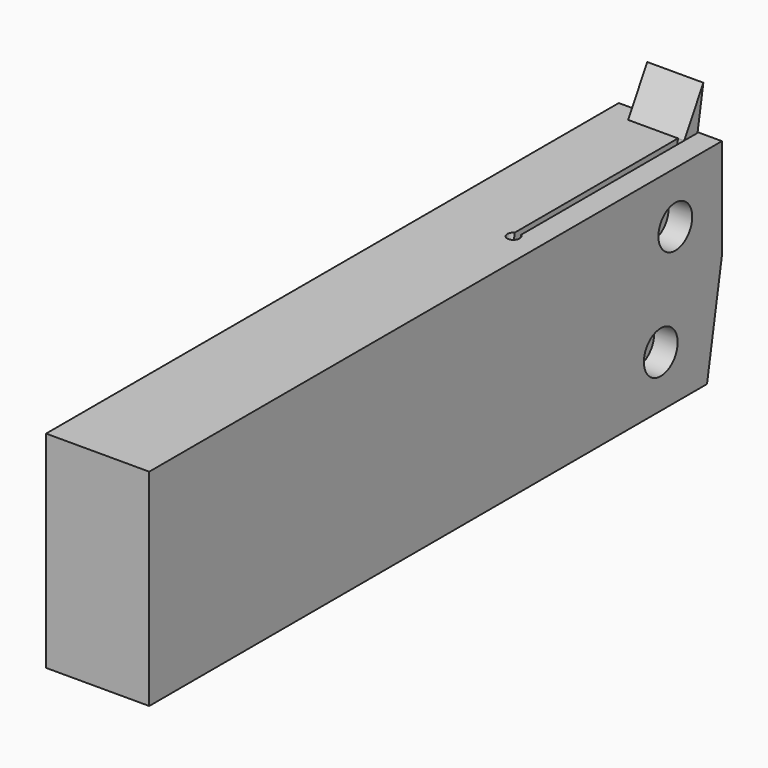
from build123d import *

# Parameters (mm, degrees)
F1_DEPTH      = 6.9088
F0_R          = 2.6
F0_R_2        = 2.1
F2_DEPTH      = 9.8044
F2_DEPTH_BACK = 2.8956
F4_DEPTH      = 31.751
F4_DEPTH_BACK = 14.4809433496
F5_R          = 2.6
F5_R_2        = 2.1
F6_DEPTH      = 3.6576


with BuildPart() as f1:
    # F0 (on Right) → F1 (new body)
    with BuildSketch(Plane.YZ):
        Polygon((7.325553628, -30.48), (11.804258938, -5.08), (9.7670606325, -5.08), (9.7479808874, -5.113047088), (5.2751026706, -30.48), align=None)
        Polygon((11.804258938, -5.08), (12.7, 0), (9.7670606325, -5.08), align=None)
        Polygon((7.1866703591, -31.2676461581), (7.325553628, -30.48), (5.2751026706, -30.48), (5.1980480634, -30.916998393), align=None)
    extrude(amount=F1_DEPTH)


with BuildPart() as f2:
    # F0 (on Right) → F2 (new body, two sides)
    with BuildSketch(Plane.YZ) as f2_sk:
        Polygon((11.938, -5.08), (11.804258938, -5.08), (7.325553628, -30.48), (9.6468188628, -30.48), (11.938, -17.486066071), align=None)
        Polygon((7.325553628, -30.48), (11.804258938, -5.08), (9.7670606325, -5.08), (9.7479808874, -5.113047088), (5.2751026706, -30.48), align=None)
        Polygon((9.7479808874, -5.113047088), (9.7670606325, -5.08), (-76.2, -5.08), (-76.2, -30.48), (5.2751026706, -30.48), align=None)
        with Locations((2.5260036068, -24.13)):
            Circle(F0_R, mode=Mode.SUBTRACT)
        with Locations((4.7653562618, -11.43)):
            Circle(F0_R, mode=Mode.SUBTRACT)
        with Locations((2.5260036068, -24.13)):
            Circle(F0_R)
        with Locations((2.5260036068, -24.13)):
            Circle(F0_R_2, mode=Mode.SUBTRACT)
        with Locations((4.7653562618, -11.43)):
            Circle(F0_R)
        with Locations((4.7653562618, -11.43)):
            Circle(F0_R_2, mode=Mode.SUBTRACT)
    extrude(amount=F2_DEPTH)
    extrude(f2_sk.sketch, amount=-F2_DEPTH_BACK)

    # F3 (on face) → F4 (cut, two sides)
    with BuildSketch(Plane(origin=(0, -5.1303777829, -29.095818248), x_dir=(1, 0, 0), z_dir=(0, -0.1736481777, -0.984807753))) as f4_sk:
        Polygon((6.1468, -10.4877584633), (0, -10.4877584633), (0, -12.4816584633), (0.2903233285, -12.5070584633), (6.6184766715, -12.5070584633), (6.9088, -12.4816584633), (6.9088, -10.4877584633), align=None)
        Polygon((6.6184766715, -12.5070584633), (0.2903233285, -12.5070584633), (2.54, -12.7038796686), (2.54, -14.7930584633), (4.3688, -14.7930584633), (4.3688, -12.7038796686), align=None)
        with BuildLine():
            Line((6.1468, 14.2523301791), (6.1468, -10.4877584633))
            Line((6.1468, -10.4877584633), (6.9088, -10.4877584633))
            Line((6.9088, -10.4877584633), (6.9088, 14.2523301791))
            ThreePointArc((6.9088, 14.2523301791), (6.5278, 15.6742415367), (6.1468, 14.2523301791))
        make_face()
    extrude(amount=-F4_DEPTH, mode=Mode.SUBTRACT)
    extrude(f4_sk.sketch, amount=F4_DEPTH_BACK, mode=Mode.SUBTRACT)

    # F5 (on face) → F6 (cut, through all)
    with BuildSketch(Plane.YZ.offset(6.1468)):
        with Locations((4.7653562618, -11.43)):
            Circle(F5_R)
        with Locations((4.7653562618, -11.43)):
            Circle(F5_R_2, mode=Mode.SUBTRACT)
        with Locations((2.5260036068, -24.13)):
            Circle(F5_R)
        with Locations((2.5260036068, -24.13)):
            Circle(F5_R_2, mode=Mode.SUBTRACT)
    extrude(amount=F6_DEPTH, mode=Mode.SUBTRACT)


solid = Compound([f1.part, f2.part])
